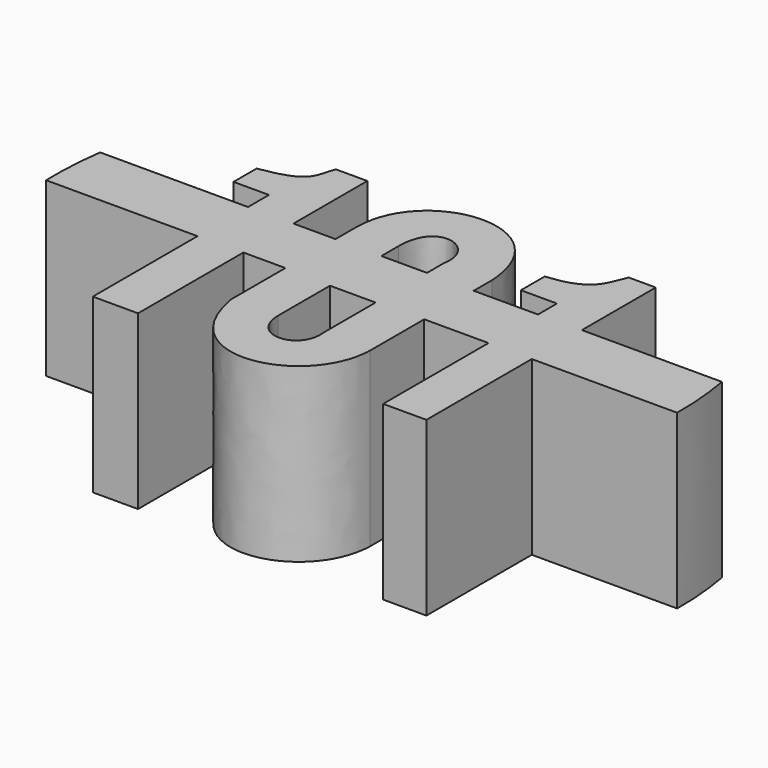
from build123d import *

# Parameters (mm, degrees)
F0_W     = 6.6796690226
F0_H     = 6.4269647701
F0_W_2   = 4.7415380832
F0_H_2   = 6.6773667932
F0_W_3   = 4.3679763669
F0_H_3   = 6.5104326932
F3_DEPTH = 17.91377


# Not quite as in the source:
# - a feature of the source that left no trace in its solid (it failed there, or was rolled back) is left out


with BuildPart() as f3:
    # F0 (on Top) → F3 (new body)
    with BuildSketch(Plane.XY):
        with BuildLine():
            Line((-7.7901906334, 10.6832636405), (-7.7901906334, 8.2267736901))
            Line((-7.7901906334, 8.2267736901), (-7.7901906334, 1.7163409969))
            Line((-7.7901906334, 1.7163409969), (-7.7901906334, -5.3760232519))
            add(Edge.make_bspline(
                [(-7.7901906334, -5.3760232519), (-5.8573922142, -16.4409913238), (6.3671558164, -13.6890839785), (6.6410573199, -5.3240084089)],
                knots=[0, 0, 0, 0, 14.4313416921, 14.4313416921, 14.4313416921, 14.4313416921], degree=3))
            Line((6.6410573199, -5.3240084089), (6.6410573199, 1.7169426428))
            Line((6.6410573199, 1.7169426428), (6.6410573199, 8.1439074129))
            Line((6.6410573199, 8.1439074129), (6.6410573199, 10.5028618127))
            add(Edge.make_bspline(
                [(-7.7901906334, 10.6832636405), (-7.9460730776, 20.2635042254), (6.0135321692, 21.5757451952), (6.6410573199, 10.5028618127)],
                knots=[0, 0, 0, 0, 14.4323754909, 14.4323754909, 14.4323754909, 14.4323754909], degree=3))
        make_face()
        with BuildLine():
            Line((-3.0246356037, 8.227375336), (-3.0246356037, 10.4858698323))
            add(Edge.make_bspline(
                [(-3.0246356037, 10.4858698323), (-2.9879831709, 15.9807316959), (2.4520969018, 14.104841277), (1.7169024795, 10.4636372998)],
                knots=[0, 0, 0, 0, 4.7415902058, 4.7415902058, 4.7415902058, 4.7415902058], degree=3))
            Line((1.7169024795, 10.4636372998), (1.7169024795, 8.227375336))
            Line((1.7169024795, 8.227375336), (1.7169024795, 1.5500085428))
            Line((1.7169024795, 1.5500085428), (1.7169024795, -5.1218802109))
            add(Edge.make_bspline(
                [(-3.0246356037, -5.2313073538), (-2.9015108012, -9.3426071107), (2.1988428198, -8.9745400473), (1.7169024795, -5.1218802109)],
                knots=[0, 0, 0, 0, 4.7428006171, 4.7428006171, 4.7428006171, 4.7428006171], degree=3))
            Line((-3.0246356037, -5.2313073538), (-3.0246356037, 1.5500085428))
            Line((-3.0246356037, 1.5500085428), (-3.0246356037, 8.227375336))
        make_face(mode=Mode.SUBTRACT)
        with BuildLine():
            add(Edge.make_bspline(
                [(-20.5391882093, 13.9101054404), (-15.6776210399, 14.6662937362), (-16.1226423563, 15.8139783774), (-15.4372690351, 17.8214814399)],
                knots=[0, 0, 0, 0, 6.4287200491, 6.4287200491, 6.4287200491, 6.4287200491], degree=3))
            Line((-20.5391882093, 13.9101054404), (-20.5391882093, 10.912990186))
            Line((-20.5391882093, 10.912990186), (-16.858519438, 10.912990186))
            Line((-16.858519438, 10.912990186), (-16.858519438, 8.1935095558))
            Line((-16.858519438, 8.1935095558), (-16.858519438, 1.6338703002))
            Line((-16.858519438, 1.6338703002), (-16.858519438, -11.9715025764))
            Line((-16.858519438, -11.9715025764), (-12.1581670002, -11.9715025764))
            Line((-12.1581670002, -11.9715025764), (-12.1581670002, 1.7163409969))
            Line((-12.1581670002, 1.7163409969), (-12.1581670002, 8.2267736901))
            Line((-12.1581670002, 8.2267736901), (-12.1581670002, 17.8214814399))
            Line((-12.1581670002, 17.8214814399), (-15.4372690351, 17.8214814399))
        make_face()
        with BuildLine():
            Line((13.3207263425, 10.6080584228), (13.3207263425, 8.1439074129))
            Line((13.3207263425, 8.1439074129), (13.3207263425, 1.7169426428))
            Line((13.3207263425, 1.7169426428), (13.3207263425, -11.9709009305))
            Line((13.3207263425, -11.9709009305), (17.8177803755, -11.9709009305))
            Line((17.8177803755, -11.9709009305), (17.8177803755, 1.7169426428))
            Line((17.8177803755, 1.7169426428), (17.8177803755, 8.227375336))
            Line((17.8177803755, 8.227375336), (17.8177803755, 17.8220830858))
            Line((17.8177803755, 17.8220830858), (15.0071214885, 17.8220830858))
            add(Edge.make_bspline(
                [(9.5731783658, 13.6997830123), (14.1142597422, 14.0927145258), (14.2135191709, 16.0034615546), (15.0071214885, 17.8220830858)],
                knots=[0, 0, 0, 0, 6.820637489, 6.820637489, 6.820637489, 6.820637489], degree=3))
            Line((9.5731783658, 13.6997830123), (9.5731783658, 10.6080584228))
            Line((9.5731783658, 10.6080584228), (13.3207263425, 10.6080584228))
        make_face()
        with BuildLine():
            Line((-16.858519438, 1.6338703002), (-16.858519438, 8.1935095558))
            Line((-16.858519438, 8.1935095558), (-32.2274787855, 8.1935095558))
            add(Edge.make_bspline(
                [(-32.2274787855, 8.1935095558), (-32.5451358574, 5.8624682682), (-32.6565323778, 3.6785873351), (-32.5981434394, 1.6338703002)],
                knots=[2.9954620198, 2.9954620198, 2.9954620198, 2.9954620198, 7.0566986479, 7.0566986479, 7.0566986479, 7.0566986479], degree=3))
            Line((-32.5981434394, 1.6338703002), (-16.858519438, 1.6338703002))
        make_face()
        with BuildLine():
            Line((17.8177803755, 1.7169426428), (32.925114671, 1.7169426428))
            add(Edge.make_bspline(
                [(32.925114671, 1.7169426428), (32.9640628967, 4.0950280506), (32.7178774406, 6.2881527237), (32.3742319383, 8.227375336)],
                knots=[25.2691995487, 25.2691995487, 25.2691995487, 25.2691995487, 32.9729040179, 32.9729040179, 32.9729040179, 32.9729040179], degree=3))
            Line((32.3742319383, 8.227375336), (17.8177803755, 8.227375336))
            Line((17.8177803755, 8.227375336), (17.8177803755, 1.7169426428))
        make_face()
        with Locations((9.9808918312, 4.9304250279)):
            Rectangle(F0_W, F0_H)
        with Locations((-0.6538665621, 4.8886919394)):
            Rectangle(F0_W_2, F0_H_2)
        with Locations((-9.9741788168, 4.9715573435)):
            Rectangle(F0_W_3, F0_H_3)
    extrude(amount=-F3_DEPTH)


solid = f3.part
